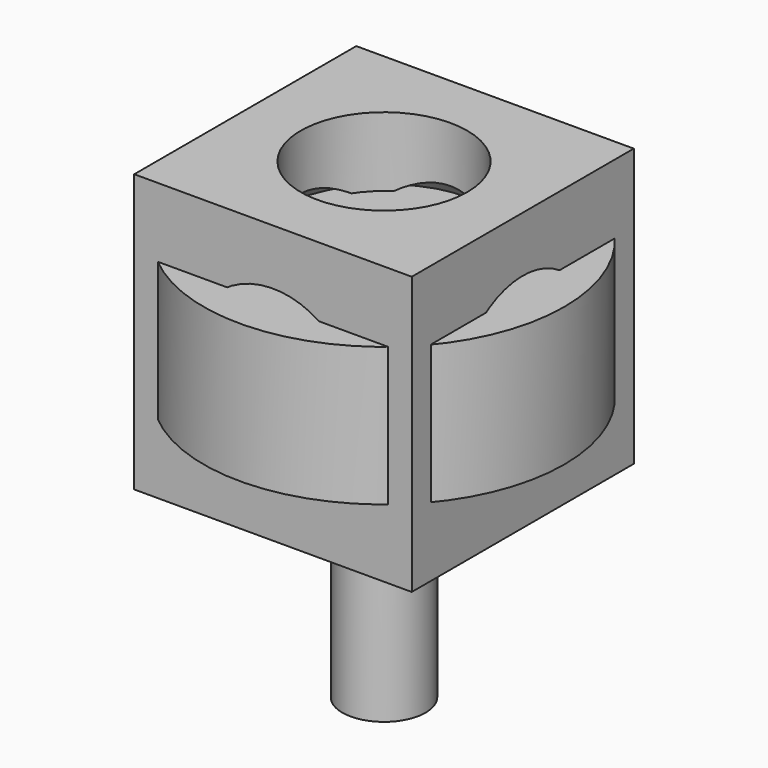
from build123d import *

# Parameters (mm, degrees)
F0_W      = 10
F0_H      = 10
F1_DEPTH  = 5
F2_R      = 3
F2_R_2    = 1.5
F3_DEPTH  = 8
F4_R      = 3
F4_R_2    = 1.5
F5_DEPTH  = 8
F6_R      = 3
F6_R_2    = 1.5
F7_DEPTH  = 8
F8_DEPTH  = 10.001
F9_DEPTH  = 10.001
F10_DEPTH = 10.001
F11_SIZE  = 1.49999
F14_R     = 6.5
F14_R_2   = 1.5
F15_DEPTH = 2.5
F16_R     = 1.5
F17_DEPTH = 1
F18_R     = 3
F18_R_2   = 1.5
F19_DEPTH = 0.25


# Not quite as in the source:
# - a fillet or chamfer is up to 0.001 mm smaller than in the source, because OpenCascade refuses the exact size


with BuildPart() as f1:
    # F0 (on Top) → F1 (new body, symmetric)
    with BuildSketch(Plane.XY):
        Rectangle(F0_W, F0_H)
    extrude(amount=F1_DEPTH, both=True)

    # F2 (on face) → F3 (cut)
    with BuildSketch(Plane.XZ.offset(5)):
        Circle(F2_R)
        Circle(F2_R_2, mode=Mode.SUBTRACT)
        Circle(F2_R_2)
    extrude(amount=-F3_DEPTH, mode=Mode.SUBTRACT)

    # F4 (on face) → F5 (cut)
    with BuildSketch(Plane.YZ.offset(5)):
        Circle(F4_R)
        Circle(F4_R_2, mode=Mode.SUBTRACT)
        Circle(F4_R_2)
    extrude(amount=-F5_DEPTH, mode=Mode.SUBTRACT)

    # F6 (on face) → F7 (cut)
    with BuildSketch(Plane.XY.offset(5)):
        Circle(F6_R)
        Circle(F6_R_2, mode=Mode.SUBTRACT)
        Circle(F6_R_2)
    extrude(amount=-F7_DEPTH, mode=Mode.SUBTRACT)

    # F2 (on face) → F8 (cut, through all)
    with BuildSketch(Plane.XZ.offset(5)):
        Circle(F2_R_2)
    extrude(amount=-F8_DEPTH, mode=Mode.SUBTRACT)

    # F4 (on face) → F9 (cut, through all)
    with BuildSketch(Plane.YZ.offset(5)):
        Circle(F4_R_2)
    extrude(amount=-F9_DEPTH, mode=Mode.SUBTRACT)

    # F6 (on face) → F10 (cut, through all)
    with BuildSketch(Plane.XY.offset(5)):
        Circle(F6_R_2)
    extrude(amount=-F10_DEPTH, mode=Mode.SUBTRACT)

    # F11 (size 1.5 in the source; OpenCascade refuses exactly that, so slightly less here)
    f11_edges = [f1.edges().sort_by_distance(p)[0] for p in [
        (-3, -1.5, 0),
        (-1.5, 3, 0),
        (-1.5, 0, -3),
    ]]
    chamfer(f11_edges, length=F11_SIZE)


with BuildPart() as f13:
    # F12 (on Front) → F13 (revolve)
    with BuildSketch(Plane.XZ):
        Polygon((0, -12), (0, 1.5), (-1.5, 1.5), (-3, 0), (-1.5, 0), (-1.5, -12), align=None)
    revolve(axis=Axis((0, 0, -5.25), (0, 0, -1)))


with BuildPart() as f15:
    # F14 (on Top) → F15 (new body, symmetric)
    with BuildSketch(Plane.XY):
        Circle(F14_R)
        Circle(F14_R_2, mode=Mode.SUBTRACT)
    extrude(amount=F15_DEPTH, both=True)


with BuildPart() as f17:
    # F16 (on Top) → F17 (new body, symmetric)
    with BuildSketch(Plane.XY):
        Polygon((2.5980762114, 1.5), (0, 3), (-2.5980762114, 1.5), (-2.5980762114, -1.5), (0, -3), (2.5980762114, -1.5), align=None)
        Circle(F16_R, mode=Mode.SUBTRACT)
    extrude(amount=F17_DEPTH, both=True)


with BuildPart() as f19:
    # F18 (on Top) → F19 (new body, symmetric)
    with BuildSketch(Plane.XY):
        Circle(F18_R)
        Circle(F18_R_2, mode=Mode.SUBTRACT)
    extrude(amount=F19_DEPTH, both=True)


solid = Compound([f1.part, f13.part, f15.part, f17.part, f19.part])
